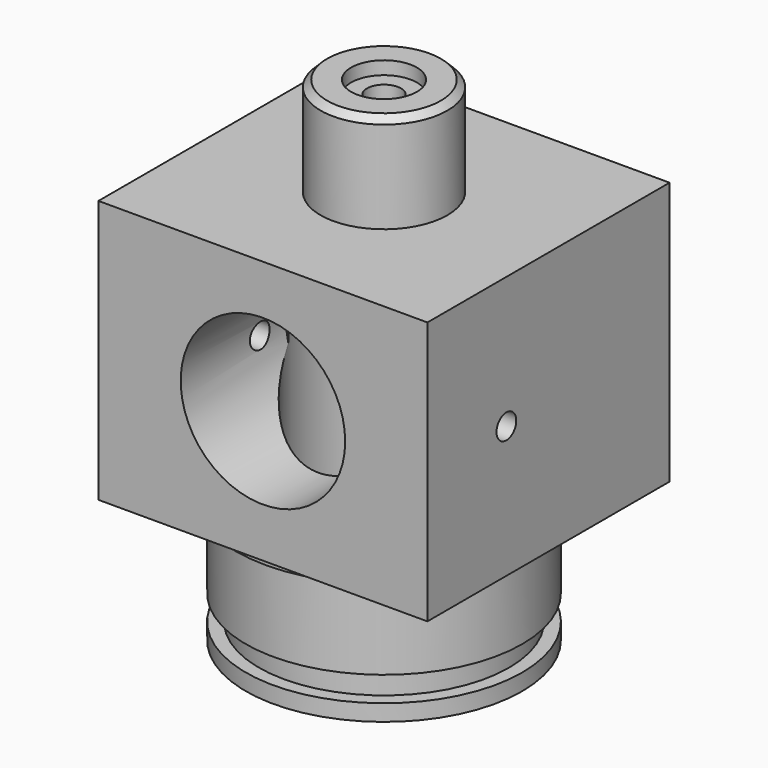
from build123d import *

# Parameters (mm, degrees)
F0_W      = 31.75
F0_H      = 29.21
F0_R      = 14.2875
F0_R_2    = 13.335
F0_R_3    = 7.9375
F0_R_4    = 1.6383
F1_DEPTH  = 25.4
F2_R      = 6.1214
F2_R_2    = 1.6383
F3_DEPTH  = 9.525
F4_R      = 3.175
F4_R_2    = 1.6383
F5_DEPTH  = 1.27
F7_DEPTH  = 21.59
F8_SIZE   = 0.635
F9_R      = 7.9375
F10_DEPTH = 12.7
F11_R     = 1.1938
F12_DEPTH = 6.35
F13_R     = 1.190625
F14_DEPTH = 31.751
F17_R     = 7.9375
F18_DEPTH = 12.7
F19_R     = 9.7155
F20_DEPTH = 0.762


# Not quite as in the source:
# - a feature names something its author has since deleted; it is built from what else it names


with BuildPart() as f1:
    # F0 (on Top) → F1 (new body)
    with BuildSketch(Plane.XY):
        Rectangle(F0_W, F0_H)
        Circle(F0_R, mode=Mode.SUBTRACT)
        Circle(F0_R)
        Circle(F0_R_2, mode=Mode.SUBTRACT)
        Circle(F0_R_2)
        Circle(F0_R_3, mode=Mode.SUBTRACT)
        Circle(F0_R_3)
        Circle(F0_R_4, mode=Mode.SUBTRACT)
    extrude(amount=F1_DEPTH)

    # F2 (on face) → F3 (join)
    with BuildSketch(Plane.XY.offset(25.4)):
        Circle(F2_R)
        Circle(F2_R_2, mode=Mode.SUBTRACT)
    extrude(amount=F3_DEPTH)

    # F4 (on face) → F5 (cut)
    with BuildSketch(Plane.XY.offset(34.925)):
        Circle(F4_R)
        Circle(F4_R_2, mode=Mode.SUBTRACT)
    extrude(amount=-F5_DEPTH, mode=Mode.SUBTRACT)

    # F0 (on Top) → F7 (cut)
    with BuildSketch(Plane.XY):
        Circle(F0_R_3)
        Circle(F0_R_4, mode=Mode.SUBTRACT)
    extrude(amount=F7_DEPTH, mode=Mode.SUBTRACT)

    # F8
    f8_edges = [f1.edges().sort_by_distance(p)[0] for p in [
        (-6.1214, 0, 34.925),
    ]]
    chamfer(f8_edges, length=F8_SIZE)

    # F9 (on face) → F10 (cut)
    with BuildSketch(Plane.XZ.offset(14.605)):
        with Locations((0, 12.7)):
            Circle(F9_R)
    extrude(amount=-F10_DEPTH, mode=Mode.SUBTRACT)

    # F11 (on face) → F12 (cut)
    with BuildSketch(Plane(origin=(0, 14.605, 0), x_dir=(-1, 0, 0), z_dir=(0, 1, 0))):
        with Locations((0, 12.7)):
            Circle(F11_R)
    extrude(amount=-F12_DEPTH, mode=Mode.SUBTRACT)

    # F13 (on face) → F14 (cut, through all)
    with BuildSketch(Plane.YZ.offset(15.875)):
        with Locations((-5.08, 12.7)):
            Circle(F13_R)
    extrude(amount=-F14_DEPTH, mode=Mode.SUBTRACT)

    # F15 (on Front) → F16 (revolve)
    with BuildSketch(Plane.XZ):
        Polygon((0, 0), (0, -12.7), (13.335, -12.7), (13.335, -11.1125), (12.065, -11.1125), (12.065, -8.6995), (13.335, -8.6995), (13.335, -0.508), (14.2875, -0.508), (14.2875, 0), align=None)
    revolve(axis=Axis((0, 0, -6.35), (0, 0, -1)))

    # F17 (on face) → F18 (cut)
    with BuildSketch(Plane(origin=(0, 0, -12.7), x_dir=(1, 0, 0), z_dir=(0, 0, -1))):
        Circle(F17_R)
    extrude(amount=-F18_DEPTH, mode=Mode.SUBTRACT)

    # F19 (on face) → F20 (cut)
    with BuildSketch(Plane(origin=(0, 0, -12.7), x_dir=(1, 0, 0), z_dir=(0, 0, -1))):
        Circle(F19_R)
    extrude(amount=-F20_DEPTH, mode=Mode.SUBTRACT)


solid = f1.part
